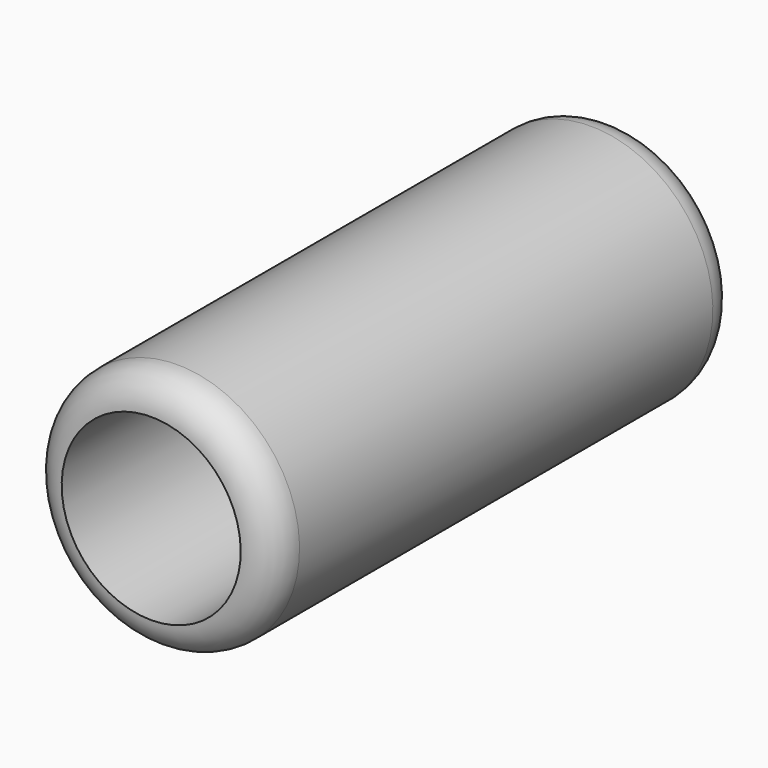
from build123d import *


# Not quite as in the source:
# - a fillet or chamfer that OpenCascade refuses, or shapes differently, is made with other operations: its cross-section is extruded or revolved along the edge and cut away or added


with BuildPart() as f1:
    # F0 (on Right) → F1 (revolve)
    with BuildSketch(Plane.YZ):
        Polygon((-59.2030874318, -23.7326024727), (54.3095125682, -23.7326024727), (54.3095125682, -6.2574024727), (50.3471125682, -6.2574024727), (50.3471125682, -17.3826024727), (-58.7138126601, -17.3826024727), align=None)
    revolve(axis=Axis((0, 27.4040363729, 0), (0, 1, 0)))

    # F2: fillet of radius 6.35 on 2 edges, made by hand

    # F2_s1 → F2_t2 (revolve, cut)
    with BuildSketch(Plane.YZ):
        with BuildLine():
            ThreePointArc((-52.3638126601, -23.7326024727), (-56.8539407206, -21.8727305333), (-58.7138126601, -17.3826024727))
            Line((-58.7138126601, -17.3826024727), (-58.8408126601, -17.3826024727))
            ThreePointArc((-58.8408126601, -17.3826024727), (-59.0850747245, -20.5478458962), (-59.3297121104, -23.7228458962))
            Line((-59.3297121104, -23.7228458962), (-59.2030874318, -23.8596024727))
            Line((-59.2030874318, -23.8596024727), (-52.3638126601, -23.8596024727))
            Line((-52.3638126601, -23.8596024727), (-52.3638126601, -23.7326024727))
        make_face()
    revolve(axis=Axis((0, -59.2030874318, 0), (0, 1, 0)), mode=Mode.SUBTRACT)

    # F2_s3 → F2_t4 (revolve, cut)
    with BuildSketch(Plane.YZ):
        with BuildLine():
            ThreePointArc((47.9595125682, -23.7326024727), (52.4496406287, -21.8727305333), (54.3095125682, -17.3826024727))
            Line((54.3095125682, -17.3826024727), (54.4365125682, -17.3826024727))
            Line((54.4365125682, -17.3826024727), (54.4365125682, -23.8596024727))
            Line((54.4365125682, -23.8596024727), (47.9595125682, -23.8596024727))
            Line((47.9595125682, -23.8596024727), (47.9595125682, -23.7326024727))
        make_face()
    revolve(axis=Axis((0, 54.3095125682, 0), (0, 1, 0)), mode=Mode.SUBTRACT)


solid = f1.part
